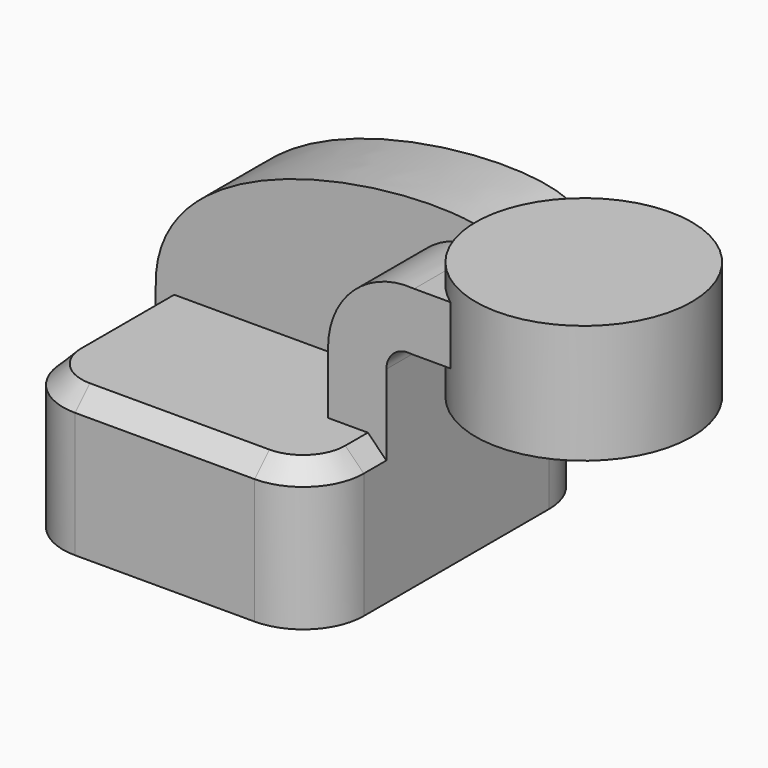
from build123d import *

# Parameters (mm, degrees)
F1_DEPTH     = 48.44446
F0_W         = 21.137111498
F0_H         = 16.0069091111
F2_DEPTH     = 24.04666
F3_DEPTH     = 24.04666
F4_DEPTH     = 15.49987
F5_DEPTH     = 16.86318
F7_R         = 16.6410292326
F8_T1_DEPTH  = 49.2679415348
F8_T3_DEPTH  = 7.7567707674
F8_T5_DEPTH  = 31.8034307674
F8_T7_DEPTH  = 7.7567707674
F8_T10_ANGLE = 90
F8_T12_ANGLE = 90
F8_T14_ANGLE = 90
F8_T16_ANGLE = 90


# Not quite as in the source:
# - a fillet or chamfer that OpenCascade refuses, or shapes differently, is made with other operations: its cross-section is extruded or revolved along the edge and cut away or added


with BuildPart() as f1:
    # F0 (on Front) → F1 (new body, symmetric)
    with BuildSketch(Plane.XZ):
        Polygon((-41.275, -19.751769717), (41.275, -19.751769717), (41.275, 19.751769717), (25.2680908889, 19.751769717), (-41.275, 19.751769717), align=None)
    extrude(amount=F1_DEPTH, both=True)

    # F0 (on Front) → F2 (join, symmetric)
    with BuildSketch(Plane.XZ):
        with BuildLine():
            Line((25.2680908889, 19.751769717), (41.275, 19.751769717))
            Line((41.275, 19.751769717), (41.275, 36.7465044527))
            ThreePointArc((41.275, 36.7465044527), (43.3382033754, 41.2513095059), (48.0968345152, 42.6317103213))
            Line((48.0968345152, 42.6317103213), (55.0704259122, 42.6317103213))
            Line((55.0704259122, 42.6317103213), (55.0704259122, 58.6386194325))
            Line((55.0704259122, 58.6386194325), (48.9036156195, 58.6386194325))
            ThreePointArc((48.9036156195, 58.6386194325), (32.3044367766, 52.8547533301), (25.2680908889, 36.7465044527))
            Line((25.2680908889, 36.7465044527), (25.2680908889, 19.751769717))
        make_face()
        with Locations((65.6389816612, 50.6351648769)):
            Rectangle(F0_W, F0_H)
        Polygon((76.2075374102, 64.215389511), (76.2075374102, 58.6386194325), (76.2075374102, 42.6317103213), (76.2075374102, 31.6205449668), (105.8704259122, 31.6205449668), (105.8704259122, 64.215389511), align=None)
    extrude(amount=F2_DEPTH, both=True)

    # F0 (on Front) → F3 (join, through all)
    with BuildSketch(Plane.XZ):
        with BuildLine():
            add(Edge.make_bspline(
                [(-41.275, 19.751769717), (-42.804622746, 65.2502314703), (54.8739225948, 71.3754703993), (55.0704259122, 58.7153048291)],
                knots=[0, 0, 0, 0, 103.688468472, 103.688468472, 103.688468472, 103.688468472], degree=3))
            Line((-41.275, 19.751769717), (25.2680908889, 19.751769717))
            Line((25.2680908889, 19.751769717), (25.2680908889, 36.7465044527))
            ThreePointArc((25.2680908889, 36.7465044527), (32.3044367766, 52.8547533301), (48.9036156195, 58.6386194325))
            Line((48.9036156195, 58.6386194325), (55.0704259122, 58.6386194325))
            Line((55.0704259122, 58.6386194325), (55.0704259122, 58.7153048291))
        make_face()
    extrude(amount=-F3_DEPTH)

    # F4 (add): a face of the model
    f4_faces = [f1.faces().sort_by_distance(p)[0] for p in [
        (105.8704259122, 0, 47.9179672389),
    ]]
    extrude(f4_faces, amount=-F4_DEPTH)

    # F5 (cut): a face of the model
    f5_faces = [f1.faces().sort_by_distance(p)[0] for p in [
        (105.8704259122, 0, 47.9179672389),
    ]]
    extrude(f5_faces, amount=-F5_DEPTH, mode=Mode.SUBTRACT)

    # F0 (on Front) → F6 (revolve)
    with BuildSketch(Plane.XZ):
        Polygon((76.2075374102, 64.215389511), (76.2075374102, 58.6386194325), (76.2075374102, 42.6317103213), (76.2075374102, 31.6205449668), (105.8704259122, 31.6205449668), (105.8704259122, 64.215389511), align=None)
    revolve(axis=Axis((76.2075374102, 0, 47.9179672389), (0, 0, 1)))

    # F7
    f7_edges = [f1.edges().sort_by_distance(p)[0] for p in [
        (-41.275, -48.44446, 0),
        (41.275, -48.44446, 0),
        (41.275, 48.44446, 0),
        (-41.275, 48.44446, 0),
    ]]
    fillet(f7_edges, radius=F7_R)

    # F8: chamfer of 5.08 on 2 edges, made by hand

    # F8_s2 → F8_t1 (cut)
    with BuildSketch(Plane.YZ.offset(-24.6339707674)):
        Polygon((43.36446, 19.751769717), (48.44446, 14.671769717), (48.44446, 19.751769717), align=None)
        Polygon((-43.36446, 19.751769717), (-48.44446, 14.671769717), (-48.44446, 19.751769717), align=None)
    extrude(amount=F8_T1_DEPTH, mode=Mode.SUBTRACT)

    # F8_s4 → F8_t3 (cut)
    with BuildSketch(Plane.XZ.offset(24.04666)):
        Polygon((36.195, 19.751769717), (41.275, 14.671769717), (41.275, 19.751769717), align=None)
    extrude(amount=F8_T3_DEPTH, mode=Mode.SUBTRACT)

    # F8_s6 → F8_t5 (cut)
    with BuildSketch(Plane.XZ):
        Polygon((-41.275, 14.671769717), (-36.195, 19.751769717), (-41.275, 19.751769717), align=None)
    extrude(amount=F8_T5_DEPTH, mode=Mode.SUBTRACT)

    # F8_s8 → F8_t7 (cut)
    with BuildSketch(Plane.XZ.offset(-31.8034307674)):
        Polygon((-41.275, 14.671769717), (-36.195, 19.751769717), (-41.275, 19.751769717), align=None)
        Polygon((36.195, 19.751769717), (41.275, 14.671769717), (41.275, 19.751769717), align=None)
    extrude(amount=F8_T7_DEPTH, mode=Mode.SUBTRACT)

    # F8_s9 → F8_t10 (revolve, cut)
    with BuildSketch(Plane.XZ.offset(31.8034307674)):
        Polygon((-41.275, 14.671769717), (-36.195, 19.751769717), (-41.275, 19.751769717), align=None)
    revolve(axis=Axis((-24.6339707674, -31.8034307674, 19.751769717), (0, 0, 1)), revolution_arc=F8_T10_ANGLE, mode=Mode.SUBTRACT)

    # F8_s11 → F8_t12 (revolve, cut)
    with BuildSketch(Plane.YZ.offset(24.6339707674)):
        Polygon((-43.36446, 19.751769717), (-48.44446, 14.671769717), (-48.44446, 19.751769717), align=None)
    revolve(axis=Axis((24.6339707674, -31.8034307674, 19.751769717), (0, 0, 1)), revolution_arc=F8_T12_ANGLE, mode=Mode.SUBTRACT)

    # F8_s13 → F8_t14 (revolve, cut)
    with BuildSketch(Plane.YZ.offset(24.6339707674)):
        Polygon((43.36446, 19.751769717), (48.44446, 14.671769717), (48.44446, 19.751769717), align=None)
    revolve(axis=Axis((24.6339707674, 31.8034307674, 19.751769717), (0, 0, -1)), revolution_arc=F8_T14_ANGLE, mode=Mode.SUBTRACT)

    # F8_s15 → F8_t16 (revolve, cut)
    with BuildSketch(Plane.XZ.offset(-31.8034307674)):
        Polygon((-41.275, 14.671769717), (-36.195, 19.751769717), (-41.275, 19.751769717), align=None)
    revolve(axis=Axis((-24.6339707674, 31.8034307674, 19.751769717), (0, 0, -1)), revolution_arc=F8_T16_ANGLE, mode=Mode.SUBTRACT)


solid = f1.part
